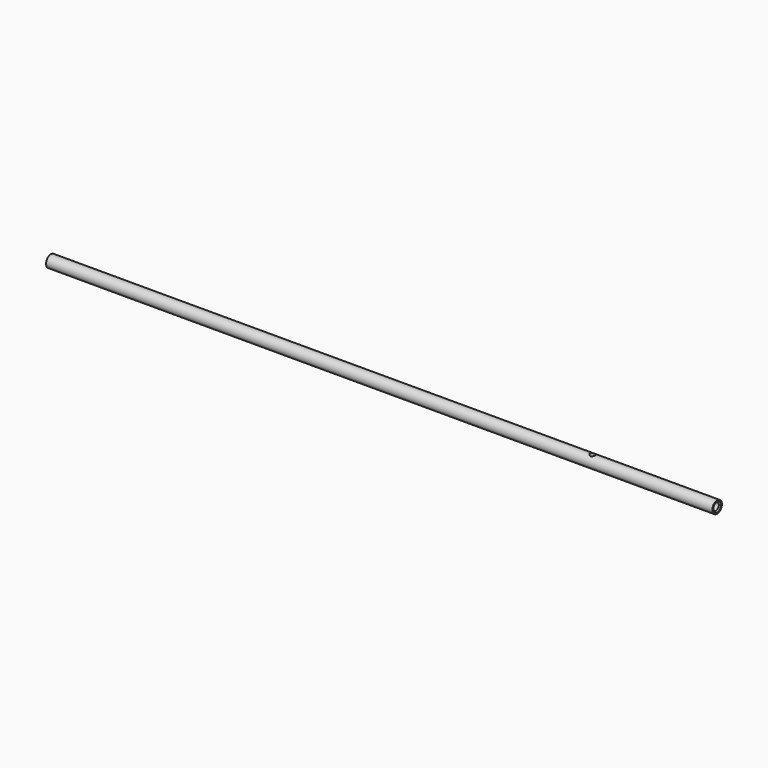
from build123d import *

# Parameters (mm, degrees)
F0_R     = 1
F1_DEPTH = 111.4
F2_W     = 2
F2_H     = 1
F3_DEPTH = 2.5
F6_R     = 0.4445
F7_DEPTH = 25


# Not quite as in the source:
# - a feature names something its author has since deleted; it is built from what else it names


with BuildPart() as f1:
    # F0 (on Right) → F1 (new body)
    with BuildSketch(Plane.YZ):
        Circle(F0_R)
    extrude(amount=F1_DEPTH)

    # F2 (on Front) → F3 (cut, symmetric)
    with BuildSketch(Plane.XZ):
        with Locations((90.6, -1.3)):
            Rectangle(F2_W, F2_H)
    extrude(amount=F3_DEPTH, both=True, mode=Mode.SUBTRACT)

    # F4 (on Front) → F5 (revolve, cut)
    with BuildSketch(Plane.XZ):
        Polygon((111.4, -0.8), (111.4, 0), (107.8, 0), (108.4, -0.6), (111.2, -0.6), align=None)
        Polygon((0.2, -0.6), (3, -0.6), (3.6, 0), (0, 0), (0, -0.8), align=None)
    revolve(axis=Axis((55.7, 0, 0), (1, 0, 0)), mode=Mode.SUBTRACT)

    # F6 (on face) → F7 (cut)
    with BuildSketch(Plane(origin=(0, 0, -0.8), x_dir=(1, 0, 0), z_dir=(0, 0, -1))):
        with Locations((90.6, 0)):
            Circle(F6_R)
    extrude(amount=-F7_DEPTH, mode=Mode.SUBTRACT)


solid = f1.part
